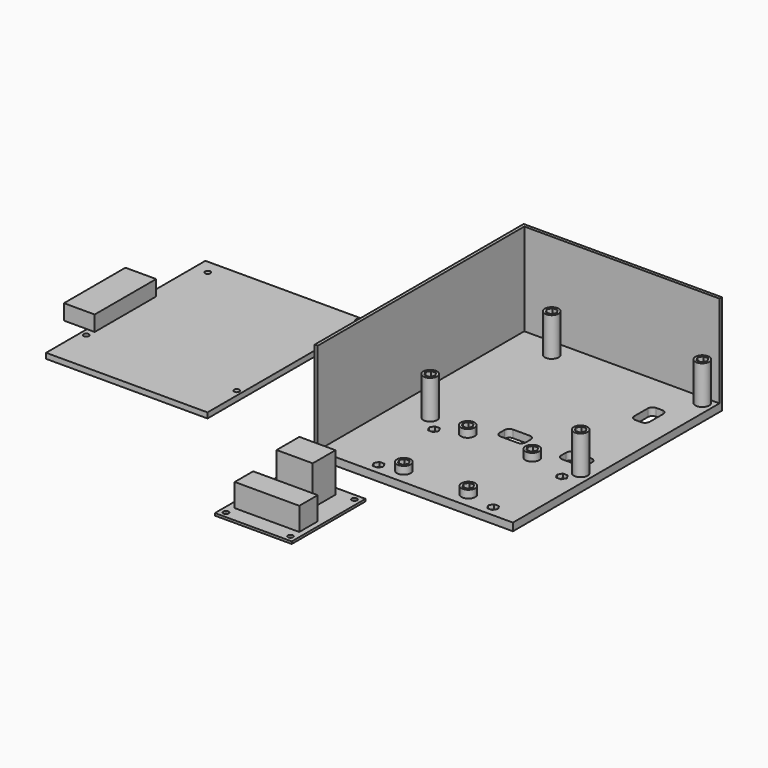
from build123d import *

# Parameters (mm, degrees)
F2_W      = 105.04
F2_H      = 129.575
F2_R      = 1.75
F3_DEPTH  = 3.5
F4_W      = 15
F4_H      = 50
F4_W_2    = 5
F5_DEPTH  = 10
F6_W      = 50
F6_H      = 60
F6_R      = 1.7
F7_DEPTH  = 1.5
F8_W      = 42
F8_H      = 15
F9_DEPTH  = 15
F10_W     = 23.5
F10_H     = 18.5
F11_DEPTH = 25.5
F12_W     = 129
F12_H     = 170
F13_DEPTH = 5
F15_D     = 3.4
F16_DEPTH = 2.8
F18_D     = 3.4
F17_R     = 4.5
F19_DEPTH = 25
F21_DEPTH = 60
F23_D     = 3.4
F22_R     = 4.5
F24_DEPTH = 5
F26_DEPTH = 10


# Not quite as in the source:
# - a feature names something its author has since deleted; it is built from what else it names


with BuildPart() as f3:
    # F2 (on Top) → F3 (new body)
    with BuildSketch(Plane.XY):
        with Locations((-122.2337017008, 64.7875)):
            Rectangle(F2_W, F2_H)
        with Locations((-170.9437017008, 27.958)):
            Circle(F2_R, mode=Mode.SUBTRACT)
        with Locations((-73.0267017008, 27.958)):
            Circle(F2_R, mode=Mode.SUBTRACT)
        with Locations((-165.8637017008, 120.414)):
            Circle(F2_R, mode=Mode.SUBTRACT)
        with Locations((-73.0267017008, 126.884)):
            Circle(F2_R, mode=Mode.SUBTRACT)
    extrude(amount=F3_DEPTH)

    # F4 (on face) → F5 (join)
    with BuildSketch(Plane.XY.offset(3.5)):
        with Locations((-182.2537017008, 58.2853868604)):
            Rectangle(F4_W, F4_H)
        with Locations((-172.2537017008, 58.2853868604)):
            Rectangle(F4_W_2, F4_H)
    extrude(amount=F5_DEPTH)


with BuildPart() as f7:
    # F6 (on Top) → F7 (new body)
    with BuildSketch(Plane.XY):
        with Locations((25, -51.1268538237)):
            Rectangle(F6_W, F6_H)
        with Locations((4, -77.1268538237)):
            Circle(F6_R, mode=Mode.SUBTRACT)
        with Locations((46, -77.1268538237)):
            Circle(F6_R, mode=Mode.SUBTRACT)
        with Locations((4, -25.1268538237)):
            Circle(F6_R, mode=Mode.SUBTRACT)
        with Locations((46, -25.1268538237)):
            Circle(F6_R, mode=Mode.SUBTRACT)
    extrude(amount=F7_DEPTH)

    # F8 (on face) → F9 (join)
    with BuildSketch(Plane.XY.offset(1.5)):
        with Locations((25.5, -63.1268538237)):
            Rectangle(F8_W, F8_H)
    extrude(amount=F9_DEPTH)

    # F10 (on face) → F11 (join)
    with BuildSketch(Plane.XY.offset(1.5)):
        with Locations((23.5, -36.3768538237)):
            Rectangle(F10_W, F10_H)
    extrude(amount=F11_DEPTH)


with BuildPart() as f13:
    # F12 (on Top) → F13 (new body)
    with BuildSketch(Plane.XY):
        with Locations((64.5, 85)):
            Rectangle(F12_W, F12_H)
    extrude(amount=F13_DEPTH)

    # F15 (through all)
    with Locations(Plane.XY.offset(5)):
        with Locations((33.5, 55.2), (116.7, 55.2), (110.5, 7), (36, 7)):
            Hole(F15_D / 2)

    # F14 (on face) → F16 (cut)
    with BuildSketch(Plane.XY.offset(5)):
        Polygon((35.1165807537, 58), (31.8834192463, 58), (30.2668384925, 55.2), (31.8834192463, 52.4), (35.1165807537, 52.4), (36.7331615075, 55.2), align=None)
        Polygon((118.3165807537, 58), (115.0834192463, 58), (113.4668384925, 55.2), (115.0834192463, 52.4), (118.3165807537, 52.4), (119.9331615075, 55.2), align=None)
        Polygon((112.1165807537, 9.8), (108.8834192463, 9.8), (107.2668384925, 7), (108.8834192463, 4.2), (112.1165807537, 4.2), (113.7331615075, 7), align=None)
        Polygon((37.6165807537, 9.8), (34.3834192463, 9.8), (32.7668384925, 7), (34.3834192463, 4.2), (37.6165807537, 4.2), (39.2331615075, 7), align=None)
    extrude(amount=-F16_DEPTH, mode=Mode.SUBTRACT)

    # F18 (through all)
    with Locations(Plane.XY.offset(5)):
        with Locations((29.08, 156.456), (121.917, 162.926), (121.917, 64), (24, 64)):
            Hole(F18_D / 2)

    # F17 (on face) → F19 (join)
    with BuildSketch(Plane.XY.offset(5)):
        with Locations((29.08, 156.456)):
            Circle(F17_R)
        Polygon((25.8468384925, 156.456), (27.4634192463, 159.256), (30.6965807537, 159.256), (32.3131615075, 156.456), (30.6965807537, 153.656), (27.4634192463, 153.656), align=None, mode=Mode.SUBTRACT)
        with Locations((121.917, 162.926)):
            Circle(F17_R)
        Polygon((118.6838384925, 162.926), (120.3004192463, 165.726), (123.5335807537, 165.726), (125.1501615075, 162.926), (123.5335807537, 160.126), (120.3004192463, 160.126), align=None, mode=Mode.SUBTRACT)
        with Locations((24, 64)):
            Circle(F17_R)
        Polygon((20.7668384925, 64), (22.3834192463, 66.8), (25.6165807537, 66.8), (27.2331615075, 64), (25.6165807537, 61.2), (22.3834192463, 61.2), align=None, mode=Mode.SUBTRACT)
        with Locations((121.917, 64)):
            Circle(F17_R)
        Polygon((118.6838384925, 64), (120.3004192463, 66.8), (123.5335807537, 66.8), (125.1501615075, 64), (123.5335807537, 61.2), (120.3004192463, 61.2), align=None, mode=Mode.SUBTRACT)
    extrude(amount=F19_DEPTH)

    # F20 (on face) → F21 (join)
    with BuildSketch(Plane.XY.offset(5)):
        Polygon((0, 170), (0, 0), (2, 0), (2, 168), (129, 168), (129, 170), align=None)
    extrude(amount=F21_DEPTH)

    # F23 (through all)
    with Locations(Plane.XY.offset(5)):
        with Locations((50, 62), (92, 62), (92, 10), (50, 10)):
            Hole(F23_D / 2)

    # F22 (on face) → F24 (join)
    with BuildSketch(Plane.XY.offset(5)):
        with Locations((50, 10)):
            Circle(F22_R)
        Polygon((46.7668384925, 10), (48.3834192463, 12.8), (51.6165807537, 12.8), (53.2331615075, 10), (51.6165807537, 7.2), (48.3834192463, 7.2), align=None, mode=Mode.SUBTRACT)
        with Locations((92, 10)):
            Circle(F22_R)
        Polygon((88.7668384925, 10), (90.3834192463, 12.8), (93.6165807537, 12.8), (95.2331615075, 10), (93.6165807537, 7.2), (90.3834192463, 7.2), align=None, mode=Mode.SUBTRACT)
        with Locations((50, 62)):
            Circle(F22_R)
        Polygon((46.7668384925, 62), (48.3834192463, 64.8), (51.6165807537, 64.8), (53.2331615075, 62), (51.6165807537, 59.2), (48.3834192463, 59.2), align=None, mode=Mode.SUBTRACT)
        with Locations((92, 62)):
            Circle(F22_R)
        Polygon((88.7668384925, 62), (90.3834192463, 64.8), (93.6165807537, 64.8), (95.2331615075, 62), (93.6165807537, 59.2), (90.3834192463, 59.2), align=None, mode=Mode.SUBTRACT)
    extrude(amount=F24_DEPTH)

    # F25 (on face) → F26 (cut)
    with BuildSketch(Plane.XY.offset(5)):
        with BuildLine():
            ThreePointArc((62, 73), (62.8786796564, 70.8786796564), (65, 70))
            Line((65, 70), (76, 70))
            ThreePointArc((76, 70), (78.1213203436, 70.8786796564), (79, 73))
            Line((79, 73), (79, 77))
            ThreePointArc((79, 77), (78.1213203436, 79.1213203436), (76, 80))
            Line((76, 80), (65, 80))
            ThreePointArc((65, 80), (62.8786796564, 79.1213203436), (62, 77))
            Line((62, 77), (62, 73))
        make_face()
        with BuildLine():
            Line((116, 80), (105, 80))
            ThreePointArc((105, 80), (102.8786796564, 79.1213203436), (102, 77))
            Line((102, 77), (102, 73))
            ThreePointArc((102, 73), (102.8786796564, 70.8786796564), (105, 70))
            Line((105, 70), (116, 70))
            ThreePointArc((116, 70), (118.1213203436, 70.8786796564), (119, 73))
            Line((119, 73), (119, 77))
            ThreePointArc((119, 77), (118.1213203436, 79.1213203436), (116, 80))
        make_face()
        with BuildLine():
            ThreePointArc((104, 130), (104.8786796564, 127.8786796564), (107, 127))
            Line((107, 127), (111, 127))
            ThreePointArc((111, 127), (113.1213203436, 127.8786796564), (114, 130))
            Line((114, 130), (114, 141))
            ThreePointArc((114, 141), (113.1213203436, 143.1213203436), (111, 144))
            Line((111, 144), (107, 144))
            ThreePointArc((107, 144), (104.8786796564, 143.1213203436), (104, 141))
            Line((104, 141), (104, 130))
        make_face()
    extrude(amount=-F26_DEPTH, mode=Mode.SUBTRACT)


solid = Compound([f3.part, f7.part, f13.part])
